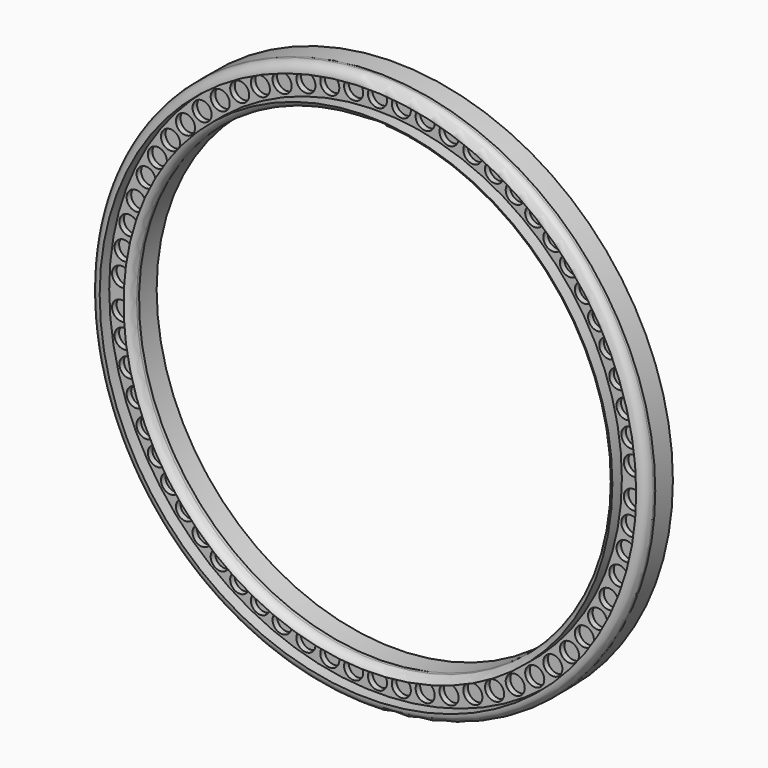
from build123d import *

# Parameters (mm, degrees)
F1_R     = 73.9775
F1_R_2   = 63.5
F2_DEPTH = 6.35
F0_R     = 73.9775
F0_R_2   = 71.4375
F0_R_3   = 65.0875
F0_R_4   = 63.5
F3_DEPTH = 3.175
F0_R_5   = 2.54
F4_DEPTH = 1.524


# Not quite as in the source:
# - a fillet or chamfer that OpenCascade refuses, or shapes differently, is made with other operations: its cross-section is extruded or revolved along the edge and cut away or added


with BuildPart() as f2:
    # F1 (on Front) → F2 (new body)
    with BuildSketch(Plane.XZ):
        with Locations((-0.3852783993, -0.2568539348)):
            Circle(F1_R)
        with Locations((-0.3852783993, -0.2568539348)):
            Circle(F1_R_2, mode=Mode.SUBTRACT)
    extrude(amount=-F2_DEPTH)

    # F0 (on Front) → F3 (join)
    with BuildSketch(Plane.XZ):
        Circle(F0_R)
        Circle(F0_R_2, mode=Mode.SUBTRACT)
        Circle(F0_R_3)
        Circle(F0_R_4, mode=Mode.SUBTRACT)
    extrude(amount=F3_DEPTH)

    # F0 (on Front) → F4 (cut)
    with BuildSketch(Plane.XZ):
        with Locations((-67.4749903807, 10.3389834788)):
            Circle(F0_R_5)
        with Locations((-66.1909868237, 16.6889834788)):
            Circle(F0_R_5)
        with Locations((-64.2570941337, 23.0389834788)):
            Circle(F0_R_5)
        with Locations((-61.6121461753, 29.3889834788)):
            Circle(F0_R_5)
        with Locations((-58.6146709728, 34.9869869095)):
            Circle(F0_R_5)
        with Locations((-55.1099839067, 40.2822365324)):
            Circle(F0_R_5)
        with Locations((-51.1284121773, 45.2289108257)):
            Circle(F0_R_5)
        with Locations((-46.7044096232, 49.7842046034)):
            Circle(F0_R_5)
        with Locations((-41.8762585813, 53.908699423)):
            Circle(F0_R_5)
        with Locations((-36.6857386172, 57.5667046856)):
            Circle(F0_R_5)
        with Locations((-31.1777649927, 60.7265664788)):
            Circle(F0_R_5)
        with Locations((-25.4, 63.360941488)):
            Circle(F0_R_5)
        with Locations((-19.05, 65.55048746)):
            Circle(F0_R_5)
        with Locations((-12.7, 67.0707008033)):
            Circle(F0_R_5)
        with Locations((-6.35, 67.9665094458)):
            Circle(F0_R_5)
        with Locations((0, 68.2625)):
            Circle(F0_R_5)
        with Locations((6.35, 67.9665094458)):
            Circle(F0_R_5)
        with Locations((12.7, 67.0707008033)):
            Circle(F0_R_5)
        with Locations((19.05, 65.55048746)):
            Circle(F0_R_5)
        with Locations((25.4, 63.360941488)):
            Circle(F0_R_5)
        with Locations((31.1777649927, 60.7265664788)):
            Circle(F0_R_5)
        with Locations((36.6857386172, 57.5667046856)):
            Circle(F0_R_5)
        with Locations((41.8762585813, 53.908699423)):
            Circle(F0_R_5)
        with Locations((46.7044096232, 49.7842046034)):
            Circle(F0_R_5)
        with Locations((51.1284121773, 45.2289108257)):
            Circle(F0_R_5)
        with Locations((55.1099839067, 40.2822365324)):
            Circle(F0_R_5)
        with Locations((58.6146709728, 34.9869869095)):
            Circle(F0_R_5)
        with Locations((61.6121461753, 29.3889834788)):
            Circle(F0_R_5)
        with Locations((64.2570941337, 23.0389834788)):
            Circle(F0_R_5)
        with Locations((66.1909868237, 16.6889834788)):
            Circle(F0_R_5)
        with Locations((67.4749903807, 10.3389834788)):
            Circle(F0_R_5)
        with Locations((68.145850329, 3.9889834788)):
            Circle(F0_R_5)
        with Locations((68.145850329, -3.9889834788)):
            Circle(F0_R_5)
        with Locations((67.4749903807, -10.3389834788)):
            Circle(F0_R_5)
        with Locations((66.1909868237, -16.6889834788)):
            Circle(F0_R_5)
        with Locations((64.2570941337, -23.0389834788)):
            Circle(F0_R_5)
        with Locations((61.6121461753, -29.3889834788)):
            Circle(F0_R_5)
        with Locations((58.6146709728, -34.9869869095)):
            Circle(F0_R_5)
        with Locations((55.1099839067, -40.2822365324)):
            Circle(F0_R_5)
        with Locations((51.1284121773, -45.2289108257)):
            Circle(F0_R_5)
        with Locations((46.7044096232, -49.7842046034)):
            Circle(F0_R_5)
        with Locations((41.8762585813, -53.908699423)):
            Circle(F0_R_5)
        with Locations((36.6857386172, -57.5667046856)):
            Circle(F0_R_5)
        with Locations((31.1777649927, -60.7265664788)):
            Circle(F0_R_5)
        with Locations((25.4, -63.360941488)):
            Circle(F0_R_5)
        with Locations((19.05, -65.55048746)):
            Circle(F0_R_5)
        with Locations((12.7, -67.0707008033)):
            Circle(F0_R_5)
        with Locations((6.35, -67.9665094458)):
            Circle(F0_R_5)
        with Locations((0, -68.2625)):
            Circle(F0_R_5)
        with Locations((-6.35, -67.9665094458)):
            Circle(F0_R_5)
        with Locations((-12.7, -67.0707008033)):
            Circle(F0_R_5)
        with Locations((-19.05, -65.55048746)):
            Circle(F0_R_5)
        with Locations((-25.4, -63.360941488)):
            Circle(F0_R_5)
        with Locations((-31.1777649927, -60.7265664788)):
            Circle(F0_R_5)
        with Locations((-36.6857386172, -57.5667046856)):
            Circle(F0_R_5)
        with Locations((-41.8762585813, -53.908699423)):
            Circle(F0_R_5)
        with Locations((-46.7044096232, -49.7842046034)):
            Circle(F0_R_5)
        with Locations((-51.1284121773, -45.2289108257)):
            Circle(F0_R_5)
        with Locations((-55.1099839067, -40.2822365324)):
            Circle(F0_R_5)
        with Locations((-58.6146709728, -34.9869869095)):
            Circle(F0_R_5)
        with Locations((-61.6121461753, -29.3889834788)):
            Circle(F0_R_5)
        with Locations((-64.2570941337, -23.0389834788)):
            Circle(F0_R_5)
        with Locations((-66.1909868237, -16.6889834788)):
            Circle(F0_R_5)
        with Locations((-67.4749903807, -10.3389834788)):
            Circle(F0_R_5)
        with Locations((-68.145850329, -3.9889834788)):
            Circle(F0_R_5)
        with Locations((-68.145850329, 3.9889834788)):
            Circle(F0_R_5)
    extrude(amount=-F4_DEPTH, mode=Mode.SUBTRACT)

    # F5: fillet of radius 2.54 on 2 edges, made by hand

    # F5_s1 → F5_t2 (revolve, cut)
    with BuildSketch(Plane.XY):
        with BuildLine():
            ThreePointArc((73.9775, -0.635), (73.2335512242, -2.4310512242), (71.4375, -3.175))
            Line((71.4375, -3.175), (73.9775, -3.175))
            Line((73.9775, -3.175), (73.9775, -0.635))
        make_face()
    revolve(axis=Axis((0, -3.175, 0), (0, -1, 0)), mode=Mode.SUBTRACT)

    # F5_s3 → F5_t4 (revolve, cut)
    with BuildSketch(Plane.XY):
        with BuildLine():
            ThreePointArc((63.5, -0.8203569803), (63.9339432581, -2.2402601461), (65.0875, -3.175))
            Line((65.0875, -3.175), (63.5, -3.175))
            Line((63.5, -3.175), (63.5, -0.8203569803))
        make_face()
    revolve(axis=Axis((0, -3.175, 0), (0, -1, 0)), mode=Mode.SUBTRACT)


solid = f2.part
